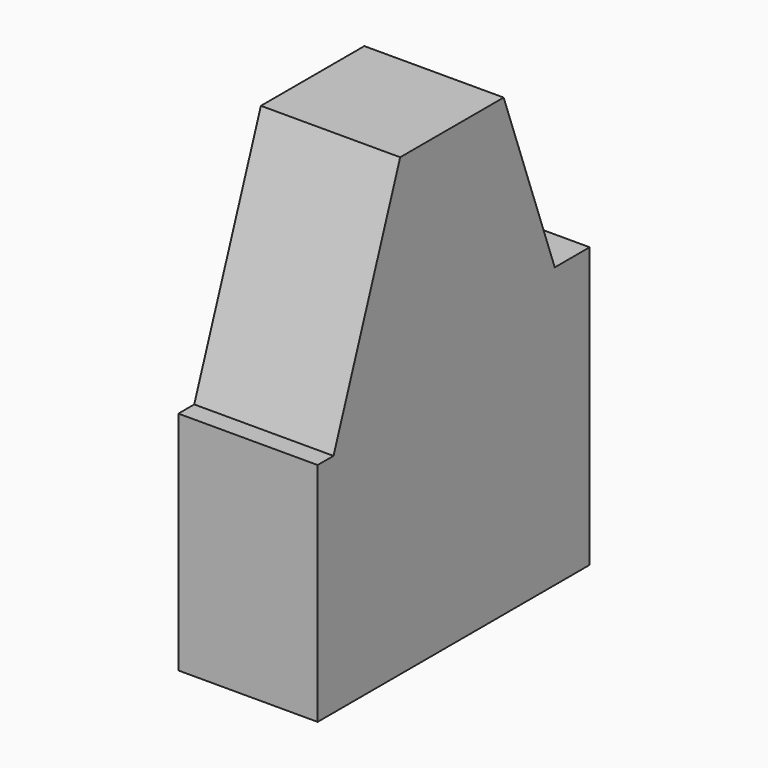
from build123d import *

# Parameters (mm, degrees)
F1_DEPTH     = 1.27
F2_W         = 1.8970449455
F2_H         = 3.5115340725
F3_DEPTH     = 1.016
F4_T4_DEPTH  = 1.8970449455
F4_T9_DEPTH  = 3.5115340725
F4_T14_DEPTH = 1.8970449455
F4_T19_DEPTH = 3.5115340725


# Not quite as in the source:
# - a fillet or chamfer that OpenCascade refuses, or shapes differently, is made with other operations: its cross-section is extruded or revolved along the edge and cut away or added


with BuildPart() as f1:
    # F0 (on Right) → F1 (new body, symmetric)
    with BuildSketch(Plane.YZ):
        Polygon((-5.8383567513, 4.1238272734), (-6.2, 4.1238272734), (-6.2, 0), (0, 0), (0, 5.1), (-0.7954361361, 5.1), (-1.9601408858, 8.3), (-4.3183541857, 8.3), align=None)
    extrude(amount=F1_DEPTH, both=True)

    # F2 (on face) → F3 (cut)
    with BuildSketch(Plane(origin=(0, 0, 0), x_dir=(-1, 0, 0), z_dir=(0, 1, 0))):
        with Locations((0, 2.7114218101)):
            Rectangle(F2_W, F2_H)
    extrude(amount=-F3_DEPTH, mode=Mode.SUBTRACT)

    # F4: chamfer of 5.08 x 0.895741062 on 4 edges, made by hand


with BuildPart() as f4_tool2:
    # F4_s3 → F4_t4 (new body)
    with BuildSketch(Plane.YZ.offset(-0.9485224728)):
        Polygon((4.064, 4.4671888463), (-1.016, 3.5714477843), (-1.016, 4.4671888463), align=None)
    extrude(amount=F4_T4_DEPTH)

    split(bisect_by=Plane.XZ, keep=Keep.TOP)


with BuildPart() as f1_1:
    add(f1.part)

    # F4_t1: union F4_tool2
    add(f4_tool2.part)


with BuildPart() as f4_tool7:
    # F4_s8 → F4_t9 (new body)
    with BuildSketch(Plane.XY.offset(4.4671888463)):
        Polygon((0.9485224728, 4.064), (0.0527814108, -1.016), (0.9485224728, -1.016), align=None)
    extrude(amount=-F4_T9_DEPTH)

    split(bisect_by=Plane.XZ, keep=Keep.TOP)


with BuildPart() as f1_2:
    add(f1_1.part)

    # F4_t6: union F4_tool7
    add(f4_tool7.part)


with BuildPart() as f4_tool12:
    # F4_s13 → F4_t14 (new body)
    with BuildSketch(Plane.YZ.offset(0.9485224728)):
        Polygon((4.064, 0.9556547739), (-1.016, 1.8513958359), (-1.016, 0.9556547739), align=None)
    extrude(amount=-F4_T14_DEPTH)

    split(bisect_by=Plane.XZ, keep=Keep.TOP)


with BuildPart() as f1_3:
    add(f1_2.part)

    # F4_t11: union F4_tool12
    add(f4_tool12.part)


with BuildPart() as f4_tool17:
    # F4_s18 → F4_t19 (new body)
    with BuildSketch(Plane.XY.offset(0.9556547739)):
        Polygon((-0.9485224728, 4.064), (-0.0527814108, -1.016), (-0.9485224728, -1.016), align=None)
    extrude(amount=F4_T19_DEPTH)

    split(bisect_by=Plane.XZ, keep=Keep.TOP)


with BuildPart() as f1_4:
    add(f1_3.part)

    # F4_t16: union F4_tool17
    add(f4_tool17.part)


solid = f1_4.part
